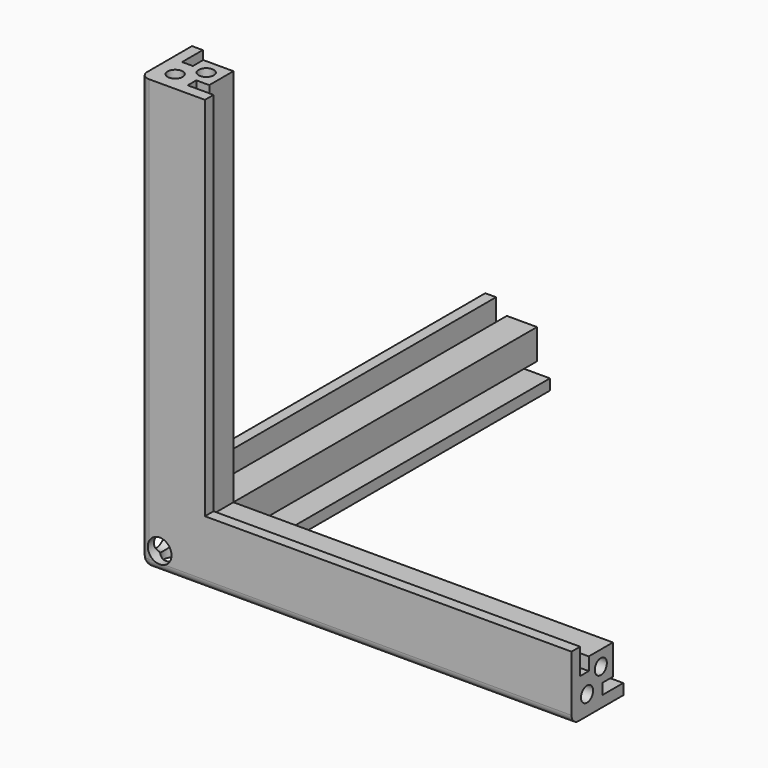
from build123d import *

# Parameters (mm, degrees)
F0_R          = 1.75
F1_DEPTH      = 100
F2_R          = 1.75
F3_DEPTH      = 100
F4_R          = 1.75
F5_DEPTH      = 100
F6_DEPTH      = 3
F7_DEPTH      = 3
F8_DEPTH      = 3
F9_R          = 2.75
F10_DEPTH     = 80
F11_R         = 2.75
F12_DEPTH     = 80
F13_R         = 2.75
F14_DEPTH     = 80
F15_T1_DEPTH  = 103
F15_T3_DEPTH  = 103
F15_T5_DEPTH  = 103
F15_S9_W      = 2
F15_S9_H      = 2
F15_T10_DEPTH = 2
F16_R         = 1.75
F17_DEPTH     = 25
F18_R         = 1.75
F19_DEPTH     = 25
F20_R         = 1.75
F21_DEPTH     = 25


# Not quite as in the source:
# - a fillet or chamfer that OpenCascade refuses, or shapes differently, is made with other operations: its cross-section is extruded or revolved along the edge and cut away or added


with BuildPart() as f1:
    # F0 (on Top) → F1 (new body)
    with BuildSketch(Plane.XY):
        Polygon((2.5, 15), (0, 15), (0, 0), (15, 0), (15, 2.5), (9, 2.5), (9, 5), (12, 5), (12, 12), (5, 12), (5, 9), (2.5, 9), align=None)
        with Locations((4.5, 4.5)):
            Circle(F0_R, mode=Mode.SUBTRACT)
    extrude(amount=F1_DEPTH)

    # F2 (on Right) → F3 (join)
    with BuildSketch(Plane.YZ):
        Polygon((2.5, 15), (0, 15), (0, 0), (15, 0), (15, 2.5), (9, 2.5), (9, 5), (12, 5), (12, 12), (5, 12), (5, 9), (2.5, 9), align=None)
        with Locations((4.5, 4.5)):
            Circle(F2_R, mode=Mode.SUBTRACT)
    extrude(amount=F3_DEPTH)

    # F4 (on Front) → F5 (join)
    with BuildSketch(Plane.XZ):
        Polygon((2.5, 15), (0, 15), (0, 0), (15, 0), (15, 2.5), (9, 2.5), (9, 5), (12, 5), (12, 12), (5, 12), (5, 9), (2.5, 9), align=None)
        with Locations((4.5, 4.5)):
            Circle(F4_R, mode=Mode.SUBTRACT)
    extrude(amount=-F5_DEPTH)

    # F6 (cut): a face of the model
    f6_faces = [f1.faces().sort_by_distance(p)[0] for p in [
        (3.75, 12, 10.5),
    ]]
    extrude(f6_faces, amount=-F6_DEPTH, mode=Mode.SUBTRACT)

    # F7 (cut): a face of the model
    f7_faces = [f1.faces().sort_by_distance(p)[0] for p in [
        (12, 3.75, 10.5),
    ]]
    extrude(f7_faces, amount=-F7_DEPTH, mode=Mode.SUBTRACT)

    # F8 (cut): a face of the model
    f8_faces = [f1.faces().sort_by_distance(p)[0] for p in [
        (12, 10.5, 3.75),
    ]]
    extrude(f8_faces, amount=-F8_DEPTH, mode=Mode.SUBTRACT)

    # F9 (on face) → F10 (cut)
    with BuildSketch(Plane(origin=(0, 0, 0), x_dir=(0, -1, 0), z_dir=(-1, 0, 0))):
        with Locations((-4.5, 4.5)):
            Circle(F9_R)
    extrude(amount=-F10_DEPTH, mode=Mode.SUBTRACT)

    # F11 (on face) → F12 (cut)
    with BuildSketch(Plane(origin=(0, 0, 0), x_dir=(1, 0, 0), z_dir=(0, 0, -1))):
        with Locations((4.5, -4.5)):
            Circle(F11_R)
    extrude(amount=-F12_DEPTH, mode=Mode.SUBTRACT)

    # F13 (on face) → F14 (cut)
    with BuildSketch(Plane.XZ):
        with Locations((4.5, 4.5)):
            Circle(F13_R)
    extrude(amount=-F14_DEPTH, mode=Mode.SUBTRACT)

    # F15: fillet of radius 2 on 3 edges, made by hand

    # F15_s2 → F15_t1 (cut)
    with BuildSketch(Plane.XZ.offset(-105)):
        with BuildLine():
            ThreePointArc((2, 0), (0.5857864376, 0.5857864376), (0, 2))
            Line((0, 2), (0, 0))
            Line((0, 0), (2, 0))
        make_face()
    extrude(amount=F15_T1_DEPTH, mode=Mode.SUBTRACT)

    # F15_s4 → F15_t3 (cut)
    with BuildSketch(Plane.YZ.offset(2)):
        with BuildLine():
            ThreePointArc((2, 0), (0.5857864376, 0.5857864376), (0, 2))
            Line((0, 2), (0, 0))
            Line((0, 0), (2, 0))
        make_face()
    extrude(amount=F15_T3_DEPTH, mode=Mode.SUBTRACT)

    # F15_s6 → F15_t5 (cut)
    with BuildSketch(Plane.XY.offset(2)):
        with BuildLine():
            ThreePointArc((2, 0), (0.5857864376, 0.5857864376), (0, 2))
            Line((0, 2), (0, 0))
            Line((0, 0), (2, 0))
        make_face()
    extrude(amount=F15_T5_DEPTH, mode=Mode.SUBTRACT)


with BuildPart() as f15_tool8:
    # F15_s9 → F15_t10 (new body)
    with BuildSketch(Plane.XY.offset(2)):
        with Locations((1, 1)):
            Rectangle(F15_S9_W, F15_S9_H)
    extrude(amount=-F15_T10_DEPTH)

    # F15_s11 → F15_t12 (revolve, cut)
    with BuildSketch(Plane(origin=(2, 2, 2), x_dir=(0.7071067812, 0.7071067812, 0), z_dir=(-0.7071067812, 0.7071067812, 0))):
        with BuildLine():
            ThreePointArc((0, -2), (2, 0), (0, 2))
            Line((0, 2), (0, -2))
        make_face()
    revolve(axis=Axis((2, 2, 2), (0, 0, -1)), mode=Mode.SUBTRACT)


with BuildPart() as f1_1:
    add(f1.part)

    # F15_t7: cut F15_tool8
    add(f15_tool8.part, mode=Mode.SUBTRACT)

    # F16 (on face) → F17 (cut)
    with BuildSketch(Plane.YZ.offset(100)):
        with Locations((8.5, 8.5)):
            Circle(F16_R)
    extrude(amount=-F17_DEPTH, mode=Mode.SUBTRACT)

    # F18 (on face) → F19 (cut)
    with BuildSketch(Plane.XY.offset(100)):
        with Locations((8.5, 8.5)):
            Circle(F18_R)
    extrude(amount=-F19_DEPTH, mode=Mode.SUBTRACT)

    # F20 (on face) → F21 (cut)
    with BuildSketch(Plane(origin=(0, 100, 0), x_dir=(-1, 0, 0), z_dir=(0, 1, 0))):
        with Locations((-8.5, 8.5)):
            Circle(F20_R)
    extrude(amount=-F21_DEPTH, mode=Mode.SUBTRACT)


solid = f1_1.part
